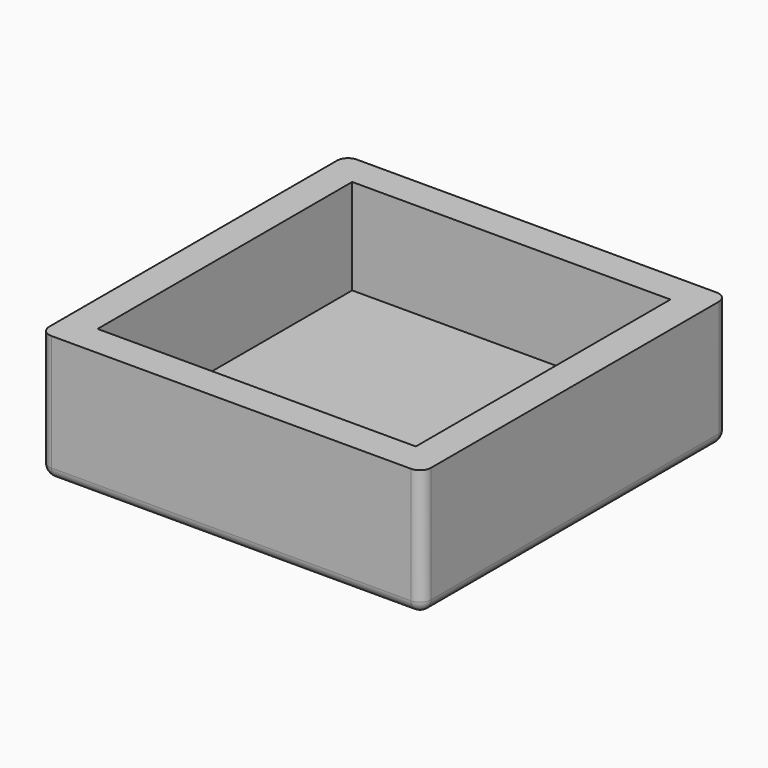
from build123d import *

# Parameters (mm, degrees)
F0_W         = 60.96
F0_H         = 60.96
F1_DEPTH     = 25.4
F2_W         = 50.8
F2_H         = 50.8
F3_DEPTH     = 20.32
F4_DEPTH     = 5.08
F5_TEXT_SIZE = 5.0411412032
F6_DEPTH     = 1.27
F7_TEXT_SIZE = 5.4371515367
F8_DEPTH     = 1.27
F9_R         = 1.778


# Not quite as in the source:
# - Text() gives the source's letters only with a copy of the font that has no kerning and outlines rounded to 1/6400 em; it was checked with that copy


with BuildPart() as f1:
    # F0 (on Top) → F1 (new body)
    with BuildSketch(Plane.XY):
        with Locations((30.48, 30.48)):
            Rectangle(F0_W, F0_H)
    extrude(amount=F1_DEPTH)

    # F2 (on face) → F3 (cut)
    with BuildSketch(Plane.XY.offset(25.4)):
        with Locations((30.48, 30.48)):
            Rectangle(F2_W, F2_H)
    extrude(amount=-F3_DEPTH, mode=Mode.SUBTRACT)

    # F4 (cut): a face of the model
    f4_faces = [f1.faces().sort_by_distance(p)[0] for p in [
        (0.8621045876, 30.48, 25.4),
    ]]
    extrude(f4_faces, amount=-F4_DEPTH, mode=Mode.SUBTRACT)

    # F5 (on face) → F6 (cut)
    with BuildSketch(Plane(origin=(0, 0, 0), x_dir=(1, 0, 0), z_dir=(0, 0, -1))):
        with Locations((11.43, -12.5793199708)):
            Text('Benjamin Child', F5_TEXT_SIZE, font='Open Sans', font_style=FontStyle.BOLD, text_align=(TextAlign.LEFT, TextAlign.BOTTOM))
    extrude(amount=-F6_DEPTH, mode=Mode.SUBTRACT)

    # F7 (on face) → F8 (cut)
    with BuildSketch(Plane(origin=(0, 0, 0), x_dir=(1, 0, 0), z_dir=(0, 0, -1))):
        with Locations((13.2290572669, -25.180766932)):
            Text('Class of 2017', F7_TEXT_SIZE, font='Open Sans', font_style=FontStyle.BOLD, text_align=(TextAlign.LEFT, TextAlign.BOTTOM))
    extrude(amount=-F8_DEPTH, mode=Mode.SUBTRACT)

    # F9
    f9_edges = [f1.edges().sort_by_distance(p)[0] for p in [
        (30.48, 0, 0),
        (0, 30.48, 0),
        (30.48, 60.96, 0),
        (60.96, 30.48, 0),
        (60.96, 60.96, 10.16),
        (0, 0, 10.16),
        (0, 60.96, 10.16),
        (60.96, 0, 10.16),
    ]]
    fillet(f9_edges, radius=F9_R)


solid = f1.part
